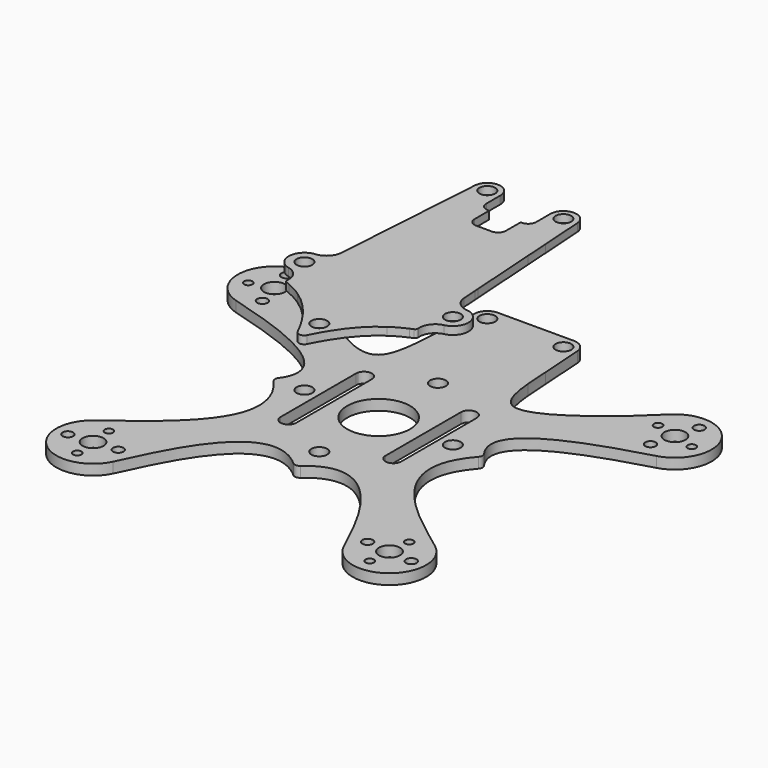
from build123d import *
from build123d import SkipClean  # not in build123d's __all__

# Parameters (mm, degrees)
F0_R     = 1
F0_R_2   = 0.8
F0_R_3   = 2
F0_R_4   = 1.5
F1_DEPTH = 2
F2_R     = 1
F4_START = 22
F4_DEPTH = 1.5
F6_DEPTH = 25
F8_R     = 1
F8_2_R   = 1


with BuildPart() as f1:
    # F0 (on Top) → F1 (new body)
    with BuildSketch(Plane.XY):
        with BuildLine():
            add(Edge.make_bspline(
                [(-33.2429738361, 26.8626836143), (-26.5641616984, 20.2477698225), (-13.0153798817, 9.5070245365), (-10.9445542744, 17.527643232), (-10.5897936727, 21.348067873)],
                knots=[0, 0, 0, 0, 0.5048386203, 0.747006273, 0.747006273, 0.747006273, 0.747006273], degree=3))
            ThreePointArc((-33.2429738361, 26.8626836143), (-44.2162134582, 25.4147755093), (-40.070061267, 15.1523270835))
            add(Edge.make_bspline(
                [(-40.070061267, 15.1523270835), (-29.4980930553, 12.1688509201), (-13.2081015036, 7.0507214405), (-20.091883092, -1)],
                knots=[0, 0, 0, 0, 25.6909570356, 25.6909570356, 25.6909570356, 25.6909570356], degree=3))
            add(Edge.make_bspline(
                [(-20.091883092, -1), (-9.2250593007, -12.2816050425), (-24.437028769, -22.0079318755), (-32.5010394378, -28.1719747319)],
                knots=[0, 0, 0, 0, 29.8714474381, 29.8714474381, 29.8714474381, 29.8714474381], degree=3))
            ThreePointArc((-32.5010394378, -28.1719747319), (-32.6879102039, -39.146734154), (-21.9629320382, -36.8111168052))
            add(Edge.make_bspline(
                [(-21.9629320382, -36.8111168052), (-19.3730118645, -31.5206269074), (-10.9737114981, -10.2415103465), (0, -21.091883092)],
                knots=[0, 0, 0, 0, 27.008604041, 27.008604041, 27.008604041, 27.008604041], degree=3))
            add(Edge.make_bspline(
                [(-8.5, -9.6630461378), (-5.1710185151, -11.9426985712), (-2.5032969266, -15.4572624153), (0, -21.091883092)],
                knots=[4.9756958029, 4.9756958029, 4.9756958029, 4.9756958029, 18.398369493, 18.398369493, 18.398369493, 18.398369493], degree=3))
            Line((-8.5, -9.6630461378), (-8.5, -10))
            ThreePointArc((-8.5, -10), (-10, -11.5), (-11.5, -10))
            Line((-11.5, -10), (-11.5, -8.0026995213))
            add(Edge.make_bspline(
                [(-12.1630677334, -7.7237885684), (-11.9392531699, -7.813530436), (-11.7182634154, -7.9064422768), (-11.5, -8.0026995213)],
                knots=[0.3902370929, 0.3902370929, 0.3902370929, 0.3902370929, 1.1728300818, 1.1728300818, 1.1728300818, 1.1728300818], degree=3))
            ThreePointArc((-12.1630677334, -7.7237885684), (-12.4001420284, -7.5260490179), (-12.4759006333, -7.2267735847))
            Line((-12.4759006333, -7.2267735847), (-12.4643353865, -7.0515581274))
            ThreePointArc((-12.4643353865, -7.0515581274), (-13.0549503284, -5.0578051119), (-14.7999785635, -3.9269852522))
            ThreePointArc((-14.7999785635, -3.9269852522), (-17.1356217405, -0.802412377), (-14.4095510697, 1.9880577269))
            ThreePointArc((-14.4095510697, 1.9880577269), (-12.5310283524, 2.8797019928), (-11.6834803989, 4.7785278308))
            Line((-11.6834803989, 4.7785278308), (-11.5, 7.5582871021))
            Line((-11.5, 7.5582871021), (-11.5, 8))
            ThreePointArc((-11.5, 8), (-11.4859484641, 8.2048344749), (-11.4440571172, 8.4058312978))
            Line((-11.4440571172, 8.4058312978), (-10.5897936727, 21.348067873))
        make_face()
        with Locations((-32.7324942237, -34.1298711871)):
            Circle(F0_R, mode=Mode.SUBTRACT)
        with Locations((-27.8754881385, -37.9667959829)):
            Circle(F0_R_2, mode=Mode.SUBTRACT)
        with Locations((-28.25, -33.7333292161)):
            Circle(F0_R_3, mode=Mode.SUBTRACT)
        with Locations((-23.7675057763, -33.3367872451)):
            Circle(F0_R, mode=Mode.SUBTRACT)
        with Locations((-28.6245118615, -29.4998624493)):
            Circle(F0_R_2, mode=Mode.SUBTRACT)
        with Locations((-42.2708443815, 20.7772989447)):
            Circle(F0_R_2, mode=Mode.SUBTRACT)
        with Locations((-39.3461816594, 26.232466033)):
            Circle(F0_R, mode=Mode.SUBTRACT)
        with Locations((-36.9915636918, 17.5459377146)):
            Circle(F0_R, mode=Mode.SUBTRACT)
        with Locations((-38.1688726756, 21.8892018738)):
            Circle(F0_R_3, mode=Mode.SUBTRACT)
        with Locations((-34.0669009697, 23.001104803)):
            Circle(F0_R_2, mode=Mode.SUBTRACT)
        with BuildLine():
            add(Edge.make_bspline(
                [(-10.5897936727, 21.348067873), (-10.4616495057, 22.7280551962), (-10.374809564, 24.267256656), (-10.2873423953, 25.9302561997)],
                knots=[0.747006273, 0.747006273, 0.747006273, 0.747006273, 0.8344803949, 0.8344803949, 0.8344803949, 0.8344803949], degree=3))
            Line((-10.5897936727, 21.348067873), (-11.4440571172, 8.4058312978))
            ThreePointArc((-11.4440571172, 8.4058312978), (-9.7951655251, 9.4859484641), (-8.5, 8))
            Line((-8.5, 8), (-8.5, -9.6630461378))
            add(Edge.make_bspline(
                [(-8.5, -9.6630461378), (-5.1710185151, -11.9426985712), (-2.5032969266, -15.4572624153), (0, -21.091883092)],
                knots=[4.9756958029, 4.9756958029, 4.9756958029, 4.9756958029, 18.398369493, 18.398369493, 18.398369493, 18.398369493], degree=3))
            Line((0, -21.091883092), (0, -16.6421356237))
            ThreePointArc((0, -16.6421356237), (-1.5, -15.1421356237), (0, -13.6421356237))
            Line((0, -13.6421356237), (0, -7))
            ThreePointArc((0, -7), (-6, -1), (0, 5))
            Line((0, 5), (0, 11.6421356237))
            ThreePointArc((0, 11.6421356237), (-1.5, 13.1421356237), (0, 14.6421356237))
            Line((0, 14.6421356237), (0, 36.4603215642))
            Line((0, 36.4603215642), (-7.2528842519, 36.4603215642))
            ThreePointArc((-7.2528842519, 36.4603215642), (-8.9353195711, 35.8094866181), (-9.7417647301, 34.1958506816))
            Line((-9.7417647301, 34.1958506816), (-10.2873423953, 25.9302561997))
        make_face()
        with Locations((-7.2528842519, 33.9603215642)):
            Circle(F0_R_4, mode=Mode.SUBTRACT)
        with BuildLine():
            Line((-11.5, -8.0026995213), (-11.5, 7.5582871021))
            Line((-11.5, 7.5582871021), (-11.6834803989, 4.7785278308))
            ThreePointArc((-11.6834803989, 4.7785278308), (-12.5310283524, 2.8797019928), (-14.4095510697, 1.9880577269))
            ThreePointArc((-14.4095510697, 1.9880577269), (-17.1356217405, -0.802412377), (-14.7999785635, -3.9269852522))
            ThreePointArc((-14.7999785635, -3.9269852522), (-13.0549503284, -5.0578051119), (-12.4643353865, -7.0515581274))
            Line((-12.4643353865, -7.0515581274), (-12.4759006333, -7.2267735847))
            ThreePointArc((-12.4759006333, -7.2267735847), (-12.4001420284, -7.5260490179), (-12.1630677334, -7.7237885684))
            add(Edge.make_bspline(
                [(-12.1630677334, -7.7237885684), (-11.9392531699, -7.813530436), (-11.7182634154, -7.9064422768), (-11.5, -8.0026995213)],
                knots=[0.3902370929, 0.3902370929, 0.3902370929, 0.3902370929, 1.1728300818, 1.1728300818, 1.1728300818, 1.1728300818], degree=3))
        make_face()
        with Locations((-14.1421356237, -1)):
            Circle(F0_R_4, mode=Mode.SUBTRACT)
    extrude(amount=F1_DEPTH)

    # F2
    f2_edges = [f1.edges().sort_by_distance(p)[0] for p in [
        (-20.091883, -1, 1),
    ]]
    fillet(f2_edges, radius=F2_R)

    # F3: F1 across face


with BuildPart() as f1_1:
    add(f1.part, clean=False)
    with SkipClean():  # cleaning this boolean's faces spoils the solid; the shape is the same uncleaned
        add(f1.part.mirror(Plane(origin=(0, 25.5512285939, 1), x_dir=(0, 1, 0), z_dir=(1, 0, 0))), clean=False)

    # F8
    f8_edges = [f1_1.edges().sort_by_distance(p)[0] for p in [
        (0, -21.091883, 1),
    ]]
    fillet(f8_edges, radius=F8_R)


with BuildPart() as f4:
    # F0 (on Top) → F4 (new body)
    with BuildSketch(Plane.XY.offset(F4_START)):
        with BuildLine():
            add(Edge.make_bspline(
                [(-10.5897936727, 21.348067873), (-10.4616495057, 22.7280551962), (-10.374809564, 24.267256656), (-10.2873423953, 25.9302561997)],
                knots=[0.747006273, 0.747006273, 0.747006273, 0.747006273, 0.8344803949, 0.8344803949, 0.8344803949, 0.8344803949], degree=3))
            Line((-10.5897936727, 21.348067873), (-11.4440571172, 8.4058312978))
            ThreePointArc((-11.4440571172, 8.4058312978), (-9.7951655251, 9.4859484641), (-8.5, 8))
            Line((-8.5, 8), (-8.5, -9.6630461378))
            add(Edge.make_bspline(
                [(-8.5, -9.6630461378), (-5.1710185151, -11.9426985712), (-2.5032969266, -15.4572624153), (0, -21.091883092)],
                knots=[4.9756958029, 4.9756958029, 4.9756958029, 4.9756958029, 18.398369493, 18.398369493, 18.398369493, 18.398369493], degree=3))
            Line((0, -21.091883092), (0, -16.6421356237))
            ThreePointArc((0, -16.6421356237), (-1.5, -15.1421356237), (0, -13.6421356237))
            Line((0, -13.6421356237), (0, -7))
            ThreePointArc((0, -7), (-6, -1), (0, 5))
            Line((0, 5), (0, 11.6421356237))
            ThreePointArc((0, 11.6421356237), (-1.5, 13.1421356237), (0, 14.6421356237))
            Line((0, 14.6421356237), (0, 36.4603215642))
            Line((0, 36.4603215642), (-7.2528842519, 36.4603215642))
            ThreePointArc((-7.2528842519, 36.4603215642), (-8.9353195711, 35.8094866181), (-9.7417647301, 34.1958506816))
            Line((-9.7417647301, 34.1958506816), (-10.2873423953, 25.9302561997))
        make_face()
        with Locations((-7.2528842519, 33.9603215642)):
            Circle(F0_R_4, mode=Mode.SUBTRACT)
        with BuildLine():
            Line((-11.5, -8.0026995213), (-11.5, 7.5582871021))
            Line((-11.5, 7.5582871021), (-11.6834803989, 4.7785278308))
            ThreePointArc((-11.6834803989, 4.7785278308), (-12.5310283524, 2.8797019928), (-14.4095510697, 1.9880577269))
            ThreePointArc((-14.4095510697, 1.9880577269), (-17.1356217405, -0.802412377), (-14.7999785635, -3.9269852522))
            ThreePointArc((-14.7999785635, -3.9269852522), (-13.0549503284, -5.0578051119), (-12.4643353865, -7.0515581274))
            Line((-12.4643353865, -7.0515581274), (-12.4759006333, -7.2267735847))
            ThreePointArc((-12.4759006333, -7.2267735847), (-12.4001420284, -7.5260490179), (-12.1630677334, -7.7237885684))
            add(Edge.make_bspline(
                [(-12.1630677334, -7.7237885684), (-11.9392531699, -7.813530436), (-11.7182634154, -7.9064422768), (-11.5, -8.0026995213)],
                knots=[0.3902370929, 0.3902370929, 0.3902370929, 0.3902370929, 1.1728300818, 1.1728300818, 1.1728300818, 1.1728300818], degree=3))
        make_face()
        with Locations((-14.1421356237, -1)):
            Circle(F0_R_4, mode=Mode.SUBTRACT)
        with BuildLine():
            ThreePointArc((-8.5, 8), (-9.7951655251, 9.4859484641), (-11.4440571172, 8.4058312978))
            Line((-11.4440571172, 8.4058312978), (-11.5, 7.5582871021))
            Line((-11.5, 7.5582871021), (-11.5, -8.0026995213))
            add(Edge.make_bspline(
                [(-11.5, -8.0026995213), (-10.4393893475, -8.4704437776), (-9.4431555789, -9.0171828549), (-8.5, -9.6630461378)],
                knots=[1.1728300818, 1.1728300818, 1.1728300818, 1.1728300818, 4.9756958029, 4.9756958029, 4.9756958029, 4.9756958029], degree=3))
            Line((-8.5, -9.6630461378), (-8.5, 8))
        make_face()
        with BuildLine():
            ThreePointArc((0, 5), (-6, -1), (0, -7))
            Line((0, -7), (0, 5))
        make_face()
        with BuildLine():
            Line((0, 11.6421356237), (0, 14.6421356237))
            ThreePointArc((0, 14.6421356237), (-1.5, 13.1421356237), (0, 11.6421356237))
        make_face()
    extrude(amount=F4_DEPTH)

    # F5 (on face) → F6 (cut)
    with BuildSketch(Plane.XY.offset(23.5)):
        with BuildLine():
            ThreePointArc((-4.7569206484, 34.1023275149), (-4.7538935548, 34.0313532165), (-4.7528842519, 33.9603215642))
            ThreePointArc((-4.7528842519, 33.9603215642), (-4.7538935548, 33.8892899118), (-4.7569206484, 33.8183156135))
            Line((-4.7569206484, 33.8183156135), (-4.7569206484, 30.6023275149))
            ThreePointArc((-4.7569206484, 30.6023275149), (-4.3175808202, 29.5416673431), (-3.2569206484, 29.1023275149))
            Line((-3.2569206484, 29.1023275149), (-3, 29.1023275149))
            Line((-3, 29.1023275149), (-3, 25.6023275149))
            ThreePointArc((-3, 25.6023275149), (-2.5606601718, 24.5416673431), (-1.5, 24.1023275149))
            Line((-1.5, 24.1023275149), (0, 24.1023275149))
            Line((0, 24.1023275149), (0, 36.4603215642))
            Line((0, 36.4603215642), (-7.2528842519, 36.4603215642))
            ThreePointArc((-7.2528842519, 36.4603215642), (-5.5360579469, 35.7776017953), (-4.7569206484, 34.1023275149))
        make_face()
    extrude(amount=-F6_DEPTH, mode=Mode.SUBTRACT)

    # F7: F4 across face


with BuildPart() as f4_1:
    add(f4.part, clean=False)
    add(f4.part.mirror(Plane(origin=(0, 5.2300959456, 22.75), x_dir=(0, 1, 0), z_dir=(1, 0, 0))), clean=False)

    # F8#2
    f8_2_edges = [f4_1.edges().sort_by_distance(p)[0] for p in [
        (0, -21.091883, 22.75),
    ]]
    fillet(f8_2_edges, radius=F8_2_R)


solid = Compound([f1_1.part, f4_1.part])
